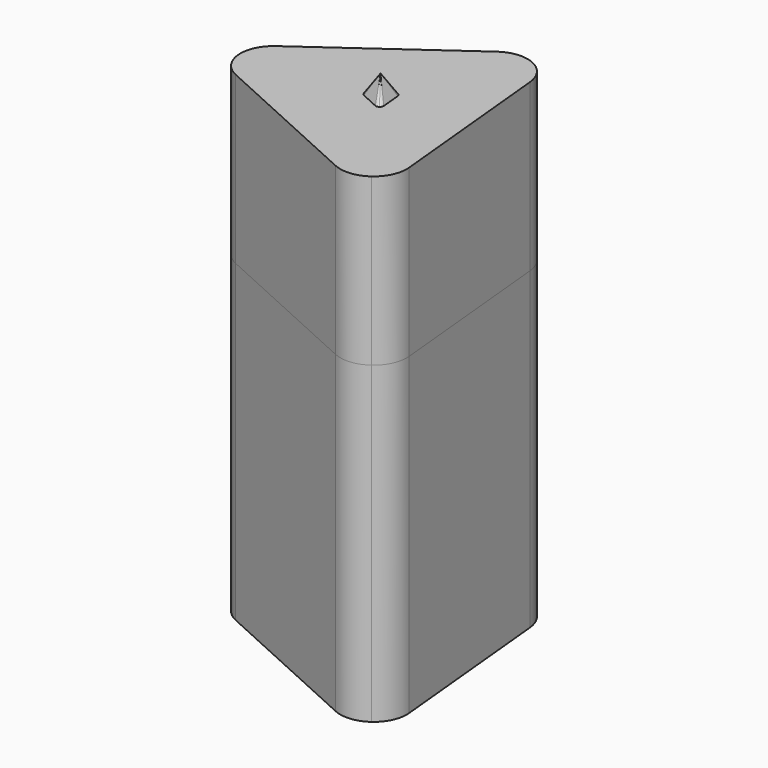
from build123d import *

# Parameters (mm, degrees)
F4_DEPTH      = 48.006
F4_DEPTH_BACK = 25.4


# Not quite as in the source:
# - a feature of the source that left no trace in its solid (it failed there, or was rolled back) is left out


with BuildPart() as f3:
    # F0 (on Top) → F3 section 0
    with BuildSketch(Plane.XY, mode=Mode.PRIVATE) as f3_s0:
        with BuildLine():
            Line((13.7612214115, -10.8844338036), (-7.7184564891, -26.2270619124))
            ThreePointArc((-7.7184564891, -26.2270619124), (-9.3897541869, -28.2572270517), (-9.8220576348, -30.8510505261))
            ThreePointArc((-9.8220576348, -30.8510505261), (-8.8995319922, -33.3135184001), (-6.8693675716, -34.9848155062))
            Line((-6.8693675716, -34.9848155062), (17.1575770817, -45.9154481789))
            ThreePointArc((17.1575770817, -45.9154481789), (19.7514000081, -46.347751922), (22.2138684317, -45.4252264958))
            ThreePointArc((22.2138684317, -45.4252264958), (23.8851659635, -43.3950617882), (24.3174697153, -40.8012388093))
            Line((24.3174697153, -40.8012388093), (21.7702029626, -14.5279780279))
            ThreePointArc((21.7702029626, -14.5279780279), (20.8476777597, -12.0655099404), (18.8175135976, -10.3942124484))
            ThreePointArc((18.8175135976, -10.3942124484), (16.2236902852, -9.9619083061), (13.7612214115, -10.8844338036))
        make_face()
    loft([f3_s0.sketch, Vertex(10.4031078517, -28.8901627064, 28.702)])


with BuildPart() as f4:
    # F0 (on Top) → F4 (new body, two sides)
    with BuildSketch(Plane.XY) as f4_sk:
        with BuildLine():
            Line((13.7612214115, -10.8844338036), (-7.7184564891, -26.2270619124))
            ThreePointArc((-7.7184564891, -26.2270619124), (-9.3897541869, -28.2572270517), (-9.8220576348, -30.8510505261))
            ThreePointArc((-9.8220576348, -30.8510505261), (-8.8995319922, -33.3135184001), (-6.8693675716, -34.9848155062))
            Line((-6.8693675716, -34.9848155062), (17.1575770817, -45.9154481789))
            ThreePointArc((17.1575770817, -45.9154481789), (19.7514000081, -46.347751922), (22.2138684317, -45.4252264958))
            ThreePointArc((22.2138684317, -45.4252264958), (23.8851659635, -43.3950617882), (24.3174697153, -40.8012388093))
            Line((24.3174697153, -40.8012388093), (21.7702029626, -14.5279780279))
            ThreePointArc((21.7702029626, -14.5279780279), (20.8476777597, -12.0655099404), (18.8175135976, -10.3942124484))
            ThreePointArc((18.8175135976, -10.3942124484), (16.2236902852, -9.9619083061), (13.7612214115, -10.8844338036))
        make_face()
    extrude(amount=-F4_DEPTH)
    extrude(f4_sk.sketch, amount=F4_DEPTH_BACK)


solid = Compound([f3.part, f4.part])
